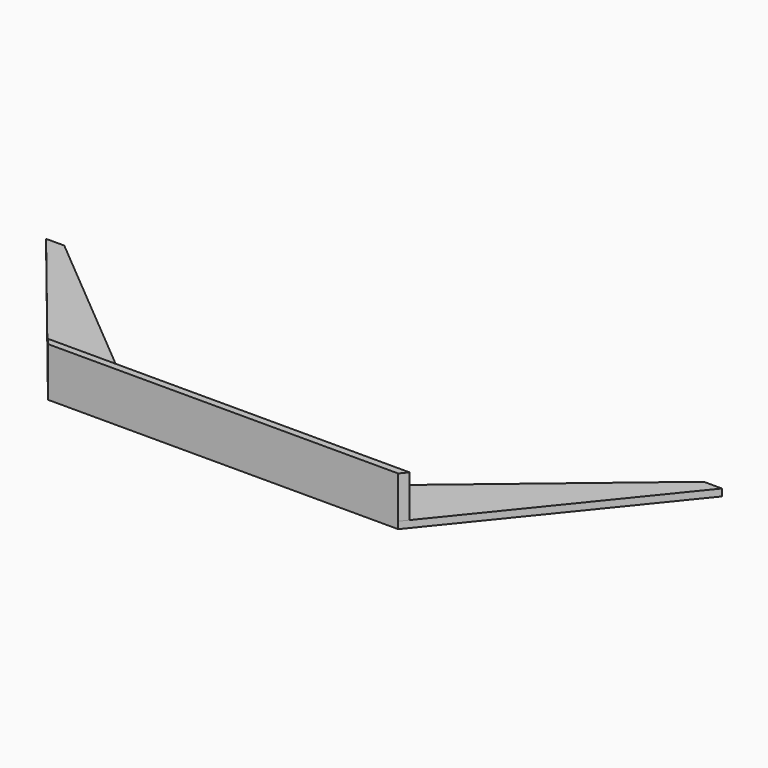
from build123d import *

# Parameters (mm, degrees)
F1_DEPTH    = 1
F3_DEPTH    = 6
F2_W        = 30
F2_H        = 2
F4_DEPTH    = 5
F5_T1_DEPTH = 40


# Not quite as in the source:
# - a fillet or chamfer that OpenCascade refuses, or shapes differently, is made with other operations: its cross-section is extruded or revolved along the edge and cut away or added


with BuildPart() as f1:
    # F0 (on Top) → F1 (new body)
    with BuildSketch(Plane.XY):
        Polygon((15, 0), (0, 0), (-15, 0), (-45.6417777248, 25.7115043875), (-48.2388163507, 25.7115043875), (-25, -3), (0, -3), (25, -3), (48.2388163507, 25.7115043875), (45.6417777248, 25.7115043875), align=None)
    extrude(amount=F1_DEPTH)

    # F2 (on face) → F3 (join)
    with BuildSketch(Plane.XY.offset(1)):
        Polygon((-15, -2), (-25.8093904115, -2), (-25, -3), (25, -3), (25.8093904115, -2), (15, -2), align=None)
    extrude(amount=F3_DEPTH)

    # F2 (on face) → F4 (join)
    with BuildSketch(Plane.XY.offset(1)):
        with Locations((0, -1)):
            Rectangle(F2_W, F2_H)
    extrude(amount=F4_DEPTH)

    # F5: fillet of radius 2 on 1 edges, made by hand

    # F5_s2 → F5_t1 (cut)
    with BuildSketch(Plane.YZ.offset(-20)):
        with BuildLine():
            add(Edge.make_bspline(
                [(0, 4), (0, 6), (-2, 6)],
                knots=[0, 0, 0, 1, 1, 1], degree=2, weights=[1, 1, 1]))
            Line((-2, 6), (0, 6))
            Line((0, 6), (0, 4))
        make_face()
    extrude(amount=F5_T1_DEPTH, mode=Mode.SUBTRACT)


solid = f1.part
